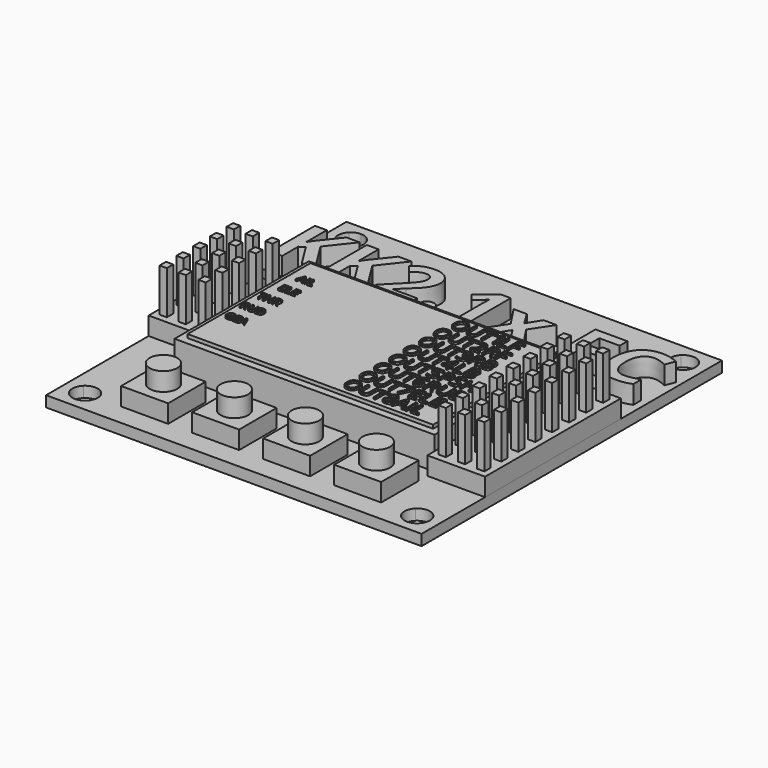
from build123d import *

# Parameters (mm, degrees)
F0_W            = 6
F0_H            = 40
F0_W_2          = 40
F0_H_2          = 6
F1_DEPTH        = 1.5
F2_W            = 36
F2_H            = 23.25
F3_DEPTH        = 4.5
F4_W            = 34
F4_H            = 21.25
F5_DEPTH        = 0.5
F6_W            = 2.6201918105
F6_H            = 2.9
F6_W_2          = 2.6899040948
F7_DEPTH        = 2.5
F6_W_3          = 2.6666666667
F6_H_2          = 2.9375
F8_W            = 1
F8_H            = 1.1067892009
F9_DEPTH        = 6
F8_H_2          = 1.1015625
F10_W           = 6.5
F10_H           = 3.25
F11_DEPTH       = 2.5
F12_R           = 1.905
F13_DEPTH       = 2.54
F14_TEXT_SIZE   = 10.8139723802
F15_DEPTH       = 2.54
F16_TEXT_SIZE   = 1.5372072234
F16_TEXT_SIZE_2 = 1.6329374936
F17_DEPTH       = 0.254
F16_TEXT_SIZE_3 = 2.6593801532
F18_DEPTH       = 0.254


# Not quite as in the source:
# - Text() gives the source's letters only with a copy of the font that has no kerning and outlines rounded to 1/6400 em; it was checked with that copy


with BuildPart() as f1:
    # F0 (on Top) → F1 (new body)
    with BuildSketch(Plane.XY):
        with Locations((25.4653038584, -3.4145421737)):
            Rectangle(F0_W, F0_H)
        with Locations((2.4653038584, -3.4145421737)):
            Rectangle(F0_W_2, F0_H)
        with Locations((2.4653038584, -26.4145421737)):
            Rectangle(F0_W_2, F0_H_2)
        with Locations((-20.5346961416, -3.4145421737)):
            Rectangle(F0_W, F0_H)
        with Locations((2.4653038584, 19.5854578263)):
            Rectangle(F0_W_2, F0_H_2)
        with BuildLine():
            Line((24.2278669913, 18.3480209592), (22.4653038584, 16.5854578263))
            Line((22.4653038584, 16.5854578263), (28.4653038584, 16.5854578263))
            Line((28.4653038584, 16.5854578263), (26.7027407254, 18.3480209592))
            ThreePointArc((26.7027407254, 18.3480209592), (25.4653038584, 17.8354578263), (24.2278669913, 18.3480209592))
        make_face()
        with BuildLine():
            Line((28.4653038584, 16.5854578263), (28.4653038584, 22.5854578263))
            Line((28.4653038584, 22.5854578263), (26.7027407254, 20.8228946934))
            ThreePointArc((26.7027407254, 20.8228946934), (27.0820930403, 20.2551538329), (27.2153038584, 19.5854578263))
            ThreePointArc((27.2153038584, 19.5854578263), (27.0820930403, 18.9157618196), (26.7027407254, 18.3480209592))
            Line((26.7027407254, 18.3480209592), (28.4653038584, 16.5854578263))
        make_face()
        with BuildLine():
            Line((28.4653038584, 22.5854578263), (22.4653038584, 22.5854578263))
            Line((22.4653038584, 22.5854578263), (24.2278669913, 20.8228946934))
            ThreePointArc((24.2278669913, 20.8228946934), (25.4653038584, 21.3354578263), (26.7027407254, 20.8228946934))
            Line((26.7027407254, 20.8228946934), (28.4653038584, 22.5854578263))
        make_face()
        with BuildLine():
            Line((24.2278669913, 20.8228946934), (22.4653038584, 22.5854578263))
            Line((22.4653038584, 22.5854578263), (22.4653038584, 16.5854578263))
            Line((22.4653038584, 16.5854578263), (24.2278669913, 18.3480209592))
            ThreePointArc((24.2278669913, 18.3480209592), (23.7153038584, 19.5854578263), (24.2278669913, 20.8228946934))
        make_face()
        with BuildLine():
            Line((28.4653038584, -29.4145421737), (28.4653038584, -23.4145421737))
            Line((28.4653038584, -23.4145421737), (26.7027407254, -25.1771053066))
            ThreePointArc((26.7027407254, -25.1771053066), (27.0820930403, -25.7448461671), (27.2153038584, -26.4145421737))
            ThreePointArc((27.2153038584, -26.4145421737), (27.0820930403, -27.0842381804), (26.7027407254, -27.6519790408))
            Line((26.7027407254, -27.6519790408), (28.4653038584, -29.4145421737))
        make_face()
        with BuildLine():
            Line((28.4653038584, -23.4145421737), (22.4653038584, -23.4145421737))
            Line((22.4653038584, -23.4145421737), (24.2278669913, -25.1771053066))
            ThreePointArc((24.2278669913, -25.1771053066), (25.4653038584, -24.6645421737), (26.7027407254, -25.1771053066))
            Line((26.7027407254, -25.1771053066), (28.4653038584, -23.4145421737))
        make_face()
        with BuildLine():
            Line((24.2278669913, -25.1771053066), (22.4653038584, -23.4145421737))
            Line((22.4653038584, -23.4145421737), (22.4653038584, -29.4145421737))
            Line((22.4653038584, -29.4145421737), (24.2278669913, -27.6519790408))
            ThreePointArc((24.2278669913, -27.6519790408), (23.7153038584, -26.4145421737), (24.2278669913, -25.1771053066))
        make_face()
        with BuildLine():
            Line((24.2278669913, -27.6519790408), (22.4653038584, -29.4145421737))
            Line((22.4653038584, -29.4145421737), (28.4653038584, -29.4145421737))
            Line((28.4653038584, -29.4145421737), (26.7027407254, -27.6519790408))
            ThreePointArc((26.7027407254, -27.6519790408), (25.4653038584, -28.1645421737), (24.2278669913, -27.6519790408))
        make_face()
        with BuildLine():
            Line((-21.7721330087, -27.6519790408), (-23.5346961416, -29.4145421737))
            Line((-23.5346961416, -29.4145421737), (-17.5346961416, -29.4145421737))
            Line((-17.5346961416, -29.4145421737), (-19.2972592746, -27.6519790408))
            ThreePointArc((-19.2972592746, -27.6519790408), (-20.5346961416, -28.1645421737), (-21.7721330087, -27.6519790408))
        make_face()
        with BuildLine():
            Line((-17.5346961416, -29.4145421737), (-17.5346961416, -23.4145421737))
            Line((-17.5346961416, -23.4145421737), (-19.2972592746, -25.1771053066))
            ThreePointArc((-19.2972592746, -25.1771053066), (-18.9179069597, -25.7448461671), (-18.7846961416, -26.4145421737))
            ThreePointArc((-18.7846961416, -26.4145421737), (-18.9179069597, -27.0842381804), (-19.2972592746, -27.6519790408))
            Line((-19.2972592746, -27.6519790408), (-17.5346961416, -29.4145421737))
        make_face()
        with BuildLine():
            Line((-17.5346961416, -23.4145421737), (-23.5346961416, -23.4145421737))
            Line((-23.5346961416, -23.4145421737), (-21.7721330087, -25.1771053066))
            ThreePointArc((-21.7721330087, -25.1771053066), (-20.5346961416, -24.6645421737), (-19.2972592746, -25.1771053066))
            Line((-19.2972592746, -25.1771053066), (-17.5346961416, -23.4145421737))
        make_face()
        with BuildLine():
            Line((-21.7721330087, -25.1771053066), (-23.5346961416, -23.4145421737))
            Line((-23.5346961416, -23.4145421737), (-23.5346961416, -29.4145421737))
            Line((-23.5346961416, -29.4145421737), (-21.7721330087, -27.6519790408))
            ThreePointArc((-21.7721330087, -27.6519790408), (-22.2846961416, -26.4145421737), (-21.7721330087, -25.1771053066))
        make_face()
        with BuildLine():
            Line((-21.7721330087, 20.8228946934), (-23.5346961416, 22.5854578263))
            Line((-23.5346961416, 22.5854578263), (-23.5346961416, 19.5854578263))
            Line((-23.5346961416, 19.5854578263), (-22.2846961416, 19.5854578263))
            ThreePointArc((-22.2846961416, 19.5854578263), (-22.1514853235, 20.2551538329), (-21.7721330087, 20.8228946934))
        make_face()
        with BuildLine():
            Line((-20.5346961416, 22.5854578263), (-23.5346961416, 22.5854578263))
            Line((-23.5346961416, 22.5854578263), (-21.7721330087, 20.8228946934))
            ThreePointArc((-21.7721330087, 20.8228946934), (-21.2043921483, 21.2022470082), (-20.5346961416, 21.3354578263))
            Line((-20.5346961416, 21.3354578263), (-20.5346961416, 22.5854578263))
        make_face()
        with BuildLine():
            Line((-17.5346961416, 22.5854578263), (-20.5346961416, 22.5854578263))
            Line((-20.5346961416, 22.5854578263), (-20.5346961416, 21.3354578263))
            ThreePointArc((-20.5346961416, 21.3354578263), (-19.865000135, 21.2022470082), (-19.2972592746, 20.8228946934))
            Line((-19.2972592746, 20.8228946934), (-17.5346961416, 22.5854578263))
        make_face()
        with BuildLine():
            Line((-17.5346961416, 16.5854578263), (-17.5346961416, 22.5854578263))
            Line((-17.5346961416, 22.5854578263), (-19.2972592746, 20.8228946934))
            ThreePointArc((-19.2972592746, 20.8228946934), (-18.9179069597, 20.2551538329), (-18.7846961416, 19.5854578263))
            ThreePointArc((-18.7846961416, 19.5854578263), (-18.9179069597, 18.9157618196), (-19.2972592746, 18.3480209592))
            Line((-19.2972592746, 18.3480209592), (-17.5346961416, 16.5854578263))
        make_face()
        with BuildLine():
            Line((-21.7721330087, 18.3480209592), (-23.5346961416, 16.5854578263))
            Line((-23.5346961416, 16.5854578263), (-17.5346961416, 16.5854578263))
            Line((-17.5346961416, 16.5854578263), (-19.2972592746, 18.3480209592))
            ThreePointArc((-19.2972592746, 18.3480209592), (-20.5346961416, 17.8354578263), (-21.7721330087, 18.3480209592))
        make_face()
        with BuildLine():
            Line((-22.2846961416, 19.5854578263), (-23.5346961416, 19.5854578263))
            Line((-23.5346961416, 19.5854578263), (-23.5346961416, 16.5854578263))
            Line((-23.5346961416, 16.5854578263), (-21.7721330087, 18.3480209592))
            ThreePointArc((-21.7721330087, 18.3480209592), (-22.1514853235, 18.9157618196), (-22.2846961416, 19.5854578263))
        make_face()
    extrude(amount=F1_DEPTH)


with BuildPart() as f3:
    # F2 (on face) → F3 (new body)
    with BuildSketch(Plane.XY.offset(1.5)):
        with Locations((2.4653038584, -5.5395421737)):
            Rectangle(F2_W, F2_H)
    extrude(amount=F3_DEPTH)


with BuildPart() as f5:
    # F4 (on face) → F5 (new body)
    with BuildSketch(Plane.XY.offset(6)):
        with Locations((2.4653038584, -5.5395421737)):
            Rectangle(F4_W, F4_H)
    extrude(amount=F5_DEPTH)


with BuildPart() as f7:
    # F6 (on face) → F7 (new body)
    with BuildSketch(Plane.XY.offset(1.5)):
        with Locations((-22.2246002364, 1.3854578263)):
            Rectangle(F6_W, F6_H)
        with Locations((-19.5695522838, 1.3854578263)):
            Rectangle(F6_W_2, F6_H)
        with Locations((-16.879648189, 1.3854578263)):
            Rectangle(F6_W_2, F6_H)
        with Locations((-16.879648189, -1.5145421737)):
            Rectangle(F6_W_2, F6_H)
        with Locations((-19.5695522838, -1.5145421737)):
            Rectangle(F6_W_2, F6_H)
        with Locations((-22.2246002364, -1.5145421737)):
            Rectangle(F6_W, F6_H)
        with Locations((-22.2246002364, -4.4145421737)):
            Rectangle(F6_W, F6_H)
        with Locations((-19.5695522838, -4.4145421737)):
            Rectangle(F6_W_2, F6_H)
        with Locations((-16.879648189, -4.4145421737)):
            Rectangle(F6_W_2, F6_H)
        with Locations((-16.879648189, -7.3145421737)):
            Rectangle(F6_W_2, F6_H)
        with Locations((-19.5695522838, -7.3145421737)):
            Rectangle(F6_W_2, F6_H)
        with Locations((-22.2246002364, -7.3145421737)):
            Rectangle(F6_W, F6_H)
        with Locations((-22.2246002364, -10.2145421737)):
            Rectangle(F6_W, F6_H)
        with Locations((-19.5695522838, -10.2145421737)):
            Rectangle(F6_W_2, F6_H)
        with Locations((-16.879648189, -10.2145421737)):
            Rectangle(F6_W_2, F6_H)
    extrude(amount=F7_DEPTH)


with BuildPart() as f7b:
    # F6 (on face) → F7, piece 2 (new body)
    with BuildSketch(Plane.XY.offset(1.5)):
        with Locations((21.7986371917, 3.6167078263)):
            Rectangle(F6_W_3, F6_H_2)
        with Locations((24.4653038584, 3.6167078263)):
            Rectangle(F6_W_3, F6_H_2)
        with Locations((27.131970525, 3.6167078263)):
            Rectangle(F6_W_3, F6_H_2)
        with Locations((27.131970525, 0.6792078263)):
            Rectangle(F6_W_3, F6_H_2)
        with Locations((24.4653038584, 0.6792078263)):
            Rectangle(F6_W_3, F6_H_2)
        with Locations((21.7986371917, 0.6792078263)):
            Rectangle(F6_W_3, F6_H_2)
        with Locations((21.7986371917, -2.2582921737)):
            Rectangle(F6_W_3, F6_H_2)
        with Locations((24.4653038584, -2.2582921737)):
            Rectangle(F6_W_3, F6_H_2)
        with Locations((27.131970525, -2.2582921737)):
            Rectangle(F6_W_3, F6_H_2)
        with Locations((27.131970525, -5.1957921737)):
            Rectangle(F6_W_3, F6_H_2)
        with Locations((24.4653038584, -5.1957921737)):
            Rectangle(F6_W_3, F6_H_2)
        with Locations((21.7986371917, -5.1957921737)):
            Rectangle(F6_W_3, F6_H_2)
        with Locations((21.7986371917, -8.1332921737)):
            Rectangle(F6_W_3, F6_H_2)
        with Locations((24.4653038584, -8.1332921737)):
            Rectangle(F6_W_3, F6_H_2)
        with Locations((27.131970525, -8.1332921737)):
            Rectangle(F6_W_3, F6_H_2)
        with Locations((27.131970525, -11.0707921737)):
            Rectangle(F6_W_3, F6_H_2)
        with Locations((24.4653038584, -11.0707921737)):
            Rectangle(F6_W_3, F6_H_2)
        with Locations((21.7986371917, -11.0707921737)):
            Rectangle(F6_W_3, F6_H_2)
        with Locations((21.7986371917, -14.0082921737)):
            Rectangle(F6_W_3, F6_H_2)
        with Locations((24.4653038584, -14.0082921737)):
            Rectangle(F6_W_3, F6_H_2)
        with Locations((27.131970525, -14.0082921737)):
            Rectangle(F6_W_3, F6_H_2)
        with Locations((27.131970525, -16.9457921737)):
            Rectangle(F6_W_3, F6_H_2)
        with Locations((24.4653038584, -16.9457921737)):
            Rectangle(F6_W_3, F6_H_2)
        Polygon((20.4653038584, -15.4770421737), (20.4653038584, -17.1645421737), (20.4653038584, -18.4145421737), (23.131970525, -18.4145421737), (23.131970525, -15.4770421737), align=None)
    extrude(amount=F7_DEPTH)


with BuildPart() as f9:
    # F8 (on face) → F9 (new body)
    with BuildSketch(Plane.XY.offset(4)):
        with Locations((-22.2246002364, 1.3854578263)):
            Rectangle(F8_W, F8_H)
    extrude(amount=F9_DEPTH)


with BuildPart() as f9b:
    # F8 (on face) → F9, piece 2 (new body)
    with BuildSketch(Plane.XY.offset(4)):
        with Locations((-19.6044084259, 1.3854578263)):
            Rectangle(F8_W, F8_H)
    extrude(amount=F9_DEPTH)


with BuildPart() as f9c:
    # F8 (on face) → F9, piece 3 (new body)
    with BuildSketch(Plane.XY.offset(4)):
        with Locations((-16.8447920469, 1.3854578263)):
            Rectangle(F8_W, F8_H)
    extrude(amount=F9_DEPTH)


with BuildPart() as f9d:
    # F8 (on face) → F9, piece 4 (new body)
    with BuildSketch(Plane.XY.offset(4)):
        with Locations((-16.8447920469, -1.5145421737)):
            Rectangle(F8_W, F8_H)
    extrude(amount=F9_DEPTH)


with BuildPart() as f9e:
    # F8 (on face) → F9, piece 5 (new body)
    with BuildSketch(Plane.XY.offset(4)):
        with Locations((-19.6044084259, -1.5145421737)):
            Rectangle(F8_W, F8_H)
    extrude(amount=F9_DEPTH)


with BuildPart() as f9f:
    # F8 (on face) → F9, piece 6 (new body)
    with BuildSketch(Plane.XY.offset(4)):
        with Locations((-22.2246002364, -1.5145421737)):
            Rectangle(F8_W, F8_H)
    extrude(amount=F9_DEPTH)


with BuildPart() as f9g:
    # F8 (on face) → F9, piece 7 (new body)
    with BuildSketch(Plane.XY.offset(4)):
        with Locations((-22.2246002364, -4.4145421737)):
            Rectangle(F8_W, F8_H)
    extrude(amount=F9_DEPTH)


with BuildPart() as f9h:
    # F8 (on face) → F9, piece 8 (new body)
    with BuildSketch(Plane.XY.offset(4)):
        with Locations((-19.6044084259, -4.4145421737)):
            Rectangle(F8_W, F8_H)
    extrude(amount=F9_DEPTH)


with BuildPart() as f9i:
    # F8 (on face) → F9, piece 9 (new body)
    with BuildSketch(Plane.XY.offset(4)):
        with Locations((-16.8447920469, -4.4145421737)):
            Rectangle(F8_W, F8_H)
    extrude(amount=F9_DEPTH)


with BuildPart() as f9j:
    # F8 (on face) → F9, piece 10 (new body)
    with BuildSketch(Plane.XY.offset(4)):
        with Locations((-16.8447920469, -7.3145421737)):
            Rectangle(F8_W, F8_H)
    extrude(amount=F9_DEPTH)


with BuildPart() as f9k:
    # F8 (on face) → F9, piece 11 (new body)
    with BuildSketch(Plane.XY.offset(4)):
        with Locations((-19.6044084259, -7.3145421737)):
            Rectangle(F8_W, F8_H)
    extrude(amount=F9_DEPTH)


with BuildPart() as f9l:
    # F8 (on face) → F9, piece 12 (new body)
    with BuildSketch(Plane.XY.offset(4)):
        with Locations((-22.2246002364, -10.2145421737)):
            Rectangle(F8_W, F8_H)
    extrude(amount=F9_DEPTH)


with BuildPart() as f9m:
    # F8 (on face) → F9, piece 13 (new body)
    with BuildSketch(Plane.XY.offset(4)):
        with Locations((-19.6044084259, -10.2145421737)):
            Rectangle(F8_W, F8_H)
    extrude(amount=F9_DEPTH)


with BuildPart() as f9n:
    # F8 (on face) → F9, piece 14 (new body)
    with BuildSketch(Plane.XY.offset(4)):
        with Locations((-16.8447920469, -10.2145421737)):
            Rectangle(F8_W, F8_H)
    extrude(amount=F9_DEPTH)


with BuildPart() as f9o:
    # F8 (on face) → F9, piece 15 (new body)
    with BuildSketch(Plane.XY.offset(4)):
        with Locations((-22.2246002364, -7.3145421737)):
            Rectangle(F8_W, F8_H)
    extrude(amount=F9_DEPTH)


with BuildPart() as f9p:
    # F8 (on face) → F9, piece 16 (new body)
    with BuildSketch(Plane.XY.offset(4)):
        with Locations((21.7986371917, 3.6167078263)):
            Rectangle(F8_W, F8_H_2)
    extrude(amount=F9_DEPTH)


with BuildPart() as f9q:
    # F8 (on face) → F9, piece 17 (new body)
    with BuildSketch(Plane.XY.offset(4)):
        with Locations((24.4653038584, 3.6167078263)):
            Rectangle(F8_W, F8_H_2)
    extrude(amount=F9_DEPTH)


with BuildPart() as f9r:
    # F8 (on face) → F9, piece 18 (new body)
    with BuildSketch(Plane.XY.offset(4)):
        with Locations((27.131970525, 3.6167078263)):
            Rectangle(F8_W, F8_H_2)
    extrude(amount=F9_DEPTH)


with BuildPart() as f9s:
    # F8 (on face) → F9, piece 19 (new body)
    with BuildSketch(Plane.XY.offset(4)):
        with Locations((27.131970525, 0.6792078263)):
            Rectangle(F8_W, F8_H_2)
    extrude(amount=F9_DEPTH)


with BuildPart() as f9t:
    # F8 (on face) → F9, piece 20 (new body)
    with BuildSketch(Plane.XY.offset(4)):
        with Locations((24.4653038584, 0.6792078263)):
            Rectangle(F8_W, F8_H_2)
    extrude(amount=F9_DEPTH)


with BuildPart() as f9u:
    # F8 (on face) → F9, piece 21 (new body)
    with BuildSketch(Plane.XY.offset(4)):
        with Locations((21.7986371917, 0.6792078263)):
            Rectangle(F8_W, F8_H_2)
    extrude(amount=F9_DEPTH)


with BuildPart() as f9v:
    # F8 (on face) → F9, piece 22 (new body)
    with BuildSketch(Plane.XY.offset(4)):
        with Locations((21.7986371917, -2.2582921737)):
            Rectangle(F8_W, F8_H_2)
    extrude(amount=F9_DEPTH)


with BuildPart() as f9w:
    # F8 (on face) → F9, piece 23 (new body)
    with BuildSketch(Plane.XY.offset(4)):
        with Locations((24.4653038584, -2.2582921737)):
            Rectangle(F8_W, F8_H_2)
    extrude(amount=F9_DEPTH)


with BuildPart() as f9x:
    # F8 (on face) → F9, piece 24 (new body)
    with BuildSketch(Plane.XY.offset(4)):
        with Locations((27.131970525, -2.2582921737)):
            Rectangle(F8_W, F8_H_2)
    extrude(amount=F9_DEPTH)


with BuildPart() as f9y:
    # F8 (on face) → F9, piece 25 (new body)
    with BuildSketch(Plane.XY.offset(4)):
        with Locations((27.131970525, -5.1957921737)):
            Rectangle(F8_W, F8_H_2)
    extrude(amount=F9_DEPTH)


with BuildPart() as f9z:
    # F8 (on face) → F9, piece 26 (new body)
    with BuildSketch(Plane.XY.offset(4)):
        with Locations((24.4653038584, -5.1957921737)):
            Rectangle(F8_W, F8_H_2)
    extrude(amount=F9_DEPTH)


with BuildPart() as f9ba:
    # F8 (on face) → F9, piece 27 (new body)
    with BuildSketch(Plane.XY.offset(4)):
        with Locations((21.7986371917, -5.1957921737)):
            Rectangle(F8_W, F8_H_2)
    extrude(amount=F9_DEPTH)


with BuildPart() as f9bb:
    # F8 (on face) → F9, piece 28 (new body)
    with BuildSketch(Plane.XY.offset(4)):
        with Locations((21.7986371917, -8.1332921737)):
            Rectangle(F8_W, F8_H_2)
    extrude(amount=F9_DEPTH)


with BuildPart() as f9bc:
    # F8 (on face) → F9, piece 29 (new body)
    with BuildSketch(Plane.XY.offset(4)):
        with Locations((24.4653038584, -8.1332921737)):
            Rectangle(F8_W, F8_H_2)
    extrude(amount=F9_DEPTH)


with BuildPart() as f9bd:
    # F8 (on face) → F9, piece 30 (new body)
    with BuildSketch(Plane.XY.offset(4)):
        with Locations((27.131970525, -8.1332921737)):
            Rectangle(F8_W, F8_H_2)
    extrude(amount=F9_DEPTH)


with BuildPart() as f9be:
    # F8 (on face) → F9, piece 31 (new body)
    with BuildSketch(Plane.XY.offset(4)):
        with Locations((27.131970525, -11.0707921737)):
            Rectangle(F8_W, F8_H_2)
    extrude(amount=F9_DEPTH)


with BuildPart() as f9bf:
    # F8 (on face) → F9, piece 32 (new body)
    with BuildSketch(Plane.XY.offset(4)):
        with Locations((24.4653038584, -11.0707921737)):
            Rectangle(F8_W, F8_H_2)
    extrude(amount=F9_DEPTH)


with BuildPart() as f9bg:
    # F8 (on face) → F9, piece 33 (new body)
    with BuildSketch(Plane.XY.offset(4)):
        with Locations((21.7986371917, -11.0707921737)):
            Rectangle(F8_W, F8_H_2)
    extrude(amount=F9_DEPTH)


with BuildPart() as f9bh:
    # F8 (on face) → F9, piece 34 (new body)
    with BuildSketch(Plane.XY.offset(4)):
        with Locations((21.7986371917, -14.0082921737)):
            Rectangle(F8_W, F8_H_2)
    extrude(amount=F9_DEPTH)


with BuildPart() as f9bi:
    # F8 (on face) → F9, piece 35 (new body)
    with BuildSketch(Plane.XY.offset(4)):
        with Locations((24.4653038584, -14.0082921737)):
            Rectangle(F8_W, F8_H_2)
    extrude(amount=F9_DEPTH)


with BuildPart() as f9bj:
    # F8 (on face) → F9, piece 36 (new body)
    with BuildSketch(Plane.XY.offset(4)):
        with Locations((27.131970525, -14.0082921737)):
            Rectangle(F8_W, F8_H_2)
    extrude(amount=F9_DEPTH)


with BuildPart() as f9bk:
    # F8 (on face) → F9, piece 37 (new body)
    with BuildSketch(Plane.XY.offset(4)):
        with Locations((27.131970525, -16.9457921737)):
            Rectangle(F8_W, F8_H_2)
    extrude(amount=F9_DEPTH)


with BuildPart() as f9bl:
    # F8 (on face) → F9, piece 38 (new body)
    with BuildSketch(Plane.XY.offset(4)):
        with Locations((24.4653038584, -16.9457921737)):
            Rectangle(F8_W, F8_H_2)
    extrude(amount=F9_DEPTH)


with BuildPart() as f9bm:
    # F8 (on face) → F9, piece 39 (new body)
    with BuildSketch(Plane.XY.offset(4)):
        with Locations((21.7986371917, -16.9457921737)):
            Rectangle(F8_W, F8_H_2)
    extrude(amount=F9_DEPTH)


with BuildPart() as f11:
    # F10 (on face) → F11 (new body)
    with BuildSketch(Plane.XY.offset(1.5)):
        with Locations((-12.2846961416, -21.5395421737)):
            Rectangle(F10_W, F10_H)
        with Locations((-12.2846961416, -24.7895421737)):
            Rectangle(F10_W, F10_H)
    extrude(amount=F11_DEPTH)


with BuildPart() as f11b:
    # F10 (on face) → F11, piece 2 (new body)
    with BuildSketch(Plane.XY.offset(1.5)):
        with Locations((-2.4513628083, -21.5395421737)):
            Rectangle(F10_W, F10_H)
        with Locations((-2.4513628083, -24.7895421737)):
            Rectangle(F10_W, F10_H)
    extrude(amount=F11_DEPTH)


with BuildPart() as f11c:
    # F10 (on face) → F11, piece 3 (new body)
    with BuildSketch(Plane.XY.offset(1.5)):
        with Locations((7.381970525, -21.5395421737)):
            Rectangle(F10_W, F10_H)
        with Locations((7.381970525, -24.7895421737)):
            Rectangle(F10_W, F10_H)
    extrude(amount=F11_DEPTH)


with BuildPart() as f11d:
    # F10 (on face) → F11, piece 4 (new body)
    with BuildSketch(Plane.XY.offset(1.5)):
        with Locations((17.2153038584, -21.5395421737)):
            Rectangle(F10_W, F10_H)
        with Locations((17.2153038584, -24.7895421737)):
            Rectangle(F10_W, F10_H)
    extrude(amount=F11_DEPTH)


with BuildPart() as f13:
    # F12 (on face) → F13 (new body)
    with BuildSketch(Plane.XY.offset(4)):
        with Locations((-12.2846961416, -23.1645421737)):
            Circle(F12_R)
    extrude(amount=F13_DEPTH)


with BuildPart() as f13b:
    # F12 (on face) → F13, piece 2 (new body)
    with BuildSketch(Plane.XY.offset(4)):
        with Locations((-2.4513628083, -23.1645421737)):
            Circle(F12_R)
    extrude(amount=F13_DEPTH)


with BuildPart() as f13c:
    # F12 (on face) → F13, piece 3 (new body)
    with BuildSketch(Plane.XY.offset(4)):
        with Locations((7.381970525, -23.1645421737)):
            Circle(F12_R)
    extrude(amount=F13_DEPTH)


with BuildPart() as f13d:
    # F12 (on face) → F13, piece 4 (new body)
    with BuildSketch(Plane.XY.offset(4)):
        with Locations((17.2153038584, -23.1645421737)):
            Circle(F12_R)
    extrude(amount=F13_DEPTH)


with BuildPart() as f15:
    # F14 (on face) → F15 (new body)
    with BuildSketch(Plane.XY.offset(1.5)):
        with Locations((-23.5346961416, 8.1953977125)):
            Text('KK2.1x FC', F14_TEXT_SIZE, font='Open Sans', font_style=FontStyle.BOLD, text_align=(TextAlign.LEFT, TextAlign.BOTTOM))
    extrude(amount=F15_DEPTH)


with BuildPart() as f17:
    # F16 (on face) → F17 (new body)
    with BuildSketch(Plane.XY.offset(6.5)):
        with Locations((-13.1691359267, 0.8320632258)):
            Text('AIL', F16_TEXT_SIZE, font='Open Sans', text_align=(TextAlign.LEFT, TextAlign.BOTTOM))
        with Locations((-13.4206134209, -2.0679367742)):
            Text('ELE', F16_TEXT_SIZE, font='Open Sans', text_align=(TextAlign.LEFT, TextAlign.BOTTOM))
        with Locations((-14.1013079946, -5.0368625687)):
            Text('THR', F16_TEXT_SIZE_2, font='Open Sans', text_align=(TextAlign.LEFT, TextAlign.BOTTOM))
        with Locations((-14.1013079946, -7.8679367742)):
            Text('RUD', F16_TEXT_SIZE, font='Open Sans', text_align=(TextAlign.LEFT, TextAlign.BOTTOM))
        with Locations((-13.9519106675, -10.7679367742)):
            Text('GEA', F16_TEXT_SIZE, font='Open Sans', text_align=(TextAlign.LEFT, TextAlign.BOTTOM))
    extrude(amount=F17_DEPTH)


with BuildPart() as f18:
    # F16 (on face) → F18 (new body)
    with BuildSketch(Plane.XY.offset(6.5)):
        with Locations((6.5362466764, 2.5115963029)):
            Text('OUT1', F16_TEXT_SIZE_3, font='Open Sans', text_align=(TextAlign.LEFT, TextAlign.BOTTOM))
        with Locations((13.1153038584, 2.5115963029)):
            Text('LF', F16_TEXT_SIZE_3, font='Open Sans', text_align=(TextAlign.LEFT, TextAlign.BOTTOM))
        with Locations((6.0866452192, -0.0622652204)):
            Text('OUT2', F16_TEXT_SIZE_3, font='Open Sans', text_align=(TextAlign.LEFT, TextAlign.BOTTOM))
        with Locations((13.1153038584, -0.0622652204)):
            Text('RF', F16_TEXT_SIZE_3, font='Open Sans', text_align=(TextAlign.LEFT, TextAlign.BOTTOM))
        with Locations((6.09994212, -2.6361267438)):
            Text('OUT3', F16_TEXT_SIZE_3, font='Open Sans', text_align=(TextAlign.LEFT, TextAlign.BOTTOM))
        with Locations((13.1153038584, -2.6361267438)):
            Text('RB', F16_TEXT_SIZE_3, font='Open Sans', text_align=(TextAlign.LEFT, TextAlign.BOTTOM))
        with Locations((5.9973066672, -5.2099882672)):
            Text('OUT4', F16_TEXT_SIZE_3, font='Open Sans', text_align=(TextAlign.LEFT, TextAlign.BOTTOM))
        with Locations((13.1153038584, -5.2099882672)):
            Text('LB', F16_TEXT_SIZE_3, font='Open Sans', text_align=(TextAlign.LEFT, TextAlign.BOTTOM))
        with Locations((6.0970334229, -7.7838497905)):
            Text('OUT5', F16_TEXT_SIZE_3, font='Open Sans', text_align=(TextAlign.LEFT, TextAlign.BOTTOM))
        with Locations((6.0737638466, -10.3577113139)):
            Text('OUT6', F16_TEXT_SIZE_3, font='Open Sans', text_align=(TextAlign.LEFT, TextAlign.BOTTOM))
        with Locations((13.1153038584, -10.3577113139)):
            Text('RUD', F16_TEXT_SIZE_3, font='Open Sans', text_align=(TextAlign.LEFT, TextAlign.BOTTOM))
        with Locations((13.1153038584, -7.7838497905)):
            Text('PSH', F16_TEXT_SIZE_3, font='Open Sans', text_align=(TextAlign.LEFT, TextAlign.BOTTOM))
        with Locations((6.0791657125, -12.9315728373)):
            Text('OUT7', F16_TEXT_SIZE_3, font='Open Sans', text_align=(TextAlign.LEFT, TextAlign.BOTTOM))
        with Locations((13.1153038584, -12.9315728373)):
            Text('ELE', F16_TEXT_SIZE_3, font='Open Sans', text_align=(TextAlign.LEFT, TextAlign.BOTTOM))
        with Locations((6.0816588814, -15.5054343606)):
            Text('OUT8', F16_TEXT_SIZE_3, font='Open Sans', text_align=(TextAlign.LEFT, TextAlign.BOTTOM))
        with Locations((13.1153038584, -15.5054343606)):
            Text('AIL', F16_TEXT_SIZE_3, font='Open Sans', text_align=(TextAlign.LEFT, TextAlign.BOTTOM))
    extrude(amount=F18_DEPTH)


solid = Compound([f1.part, f3.part, f5.part, f7.part, f7b.part, f9.part, f9b.part, f9c.part, f9d.part, f9e.part, f9f.part, f9g.part, f9h.part, f9i.part, f9j.part, f9k.part, f9l.part, f9m.part, f9n.part, f9o.part, f9p.part, f9q.part, f9r.part, f9s.part, f9t.part, f9u.part, f9v.part, f9w.part, f9x.part, f9y.part, f9z.part, f9ba.part, f9bb.part, f9bc.part, f9bd.part, f9be.part, f9bf.part, f9bg.part, f9bh.part, f9bi.part, f9bj.part, f9bk.part, f9bl.part, f9bm.part, f11.part, f11b.part, f11c.part, f11d.part, f13.part, f13b.part, f13c.part, f13d.part, f15.part, f17.part, f18.part])
